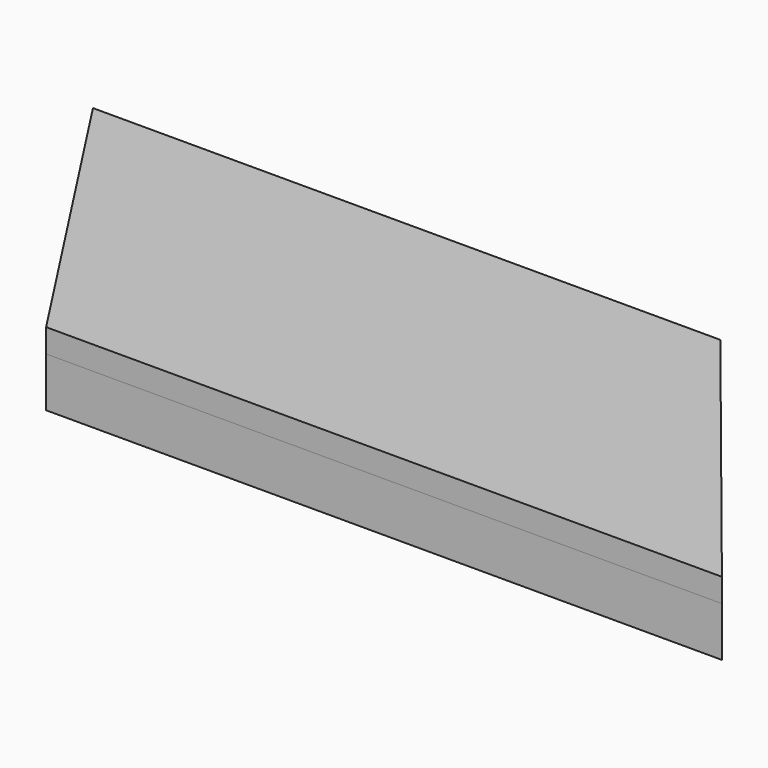
from build123d import *

# Parameters (mm, degrees)
F1_DEPTH = 2.54
F2_DEPTH = 2.794
F5_DEPTH = 2.54


# Not quite as in the source:
# - ends of sketch curves that miss each other by under 0.0002 mm in the source are joined


with BuildPart() as f1:
    # F0 (on Top) → F1 (new body)
    with BuildSketch(Plane.XY):
        Polygon((40.704589831, -14.0446320264), (45.6521262704, -14.1146421426), (31.6115576886, 3.3264026483), (26.7203815156, 3.3264026483), (24.2085343305, 6.4465921843), (-38.9784165732, 6.4465921843), (-22.1132018277, -19.5065848529), (45.1016274707, -19.5065848529), (43.1621550999, -17.0973931503), align=None)
        Polygon((26.7203815156, 3.3264026483), (31.6115576886, 3.3264026483), (26.0325449788, 10.2565921843), (-41.4542779326, 10.2565921843), (-38.9784165732, 6.4465921843), (24.2085343305, 6.4465921843), align=None)
        Polygon((53.0599689064, -23.3165845275), (49.0268522152, -18.3066903858), (45.6521262704, -14.1146421426), (40.704589831, -14.0446320264), (43.1621550999, -17.0973931503), (45.1016274707, -19.5065848529), (-22.1132018277, -19.5065848529), (-19.6373406798, -23.3165845275), align=None)
    extrude(amount=-F1_DEPTH)

    # F0 (on Top) → F2 (join)
    with BuildSketch(Plane.XY):
        Polygon((26.7203815156, 3.3264026483), (31.6115576886, 3.3264026483), (26.0325449788, 10.2565921843), (-41.4542779326, 10.2565921843), (-38.9784165732, 6.4465921843), (24.2085343305, 6.4465921843), align=None)
        Polygon((53.0599689064, -23.3165845275), (49.0268522152, -18.3066903858), (45.6521262704, -14.1146421426), (40.704589831, -14.0446320264), (43.1621550999, -17.0973931503), (45.1016274707, -19.5065848529), (-22.1132018277, -19.5065848529), (-19.6373406798, -23.3165845275), align=None)
    extrude(amount=F2_DEPTH)

    # F4 (on offset) → F5 (join)
    with BuildSketch(Plane.XY.offset(2.794)):
        Polygon((53.0598776368, -23.3175773174), (49.0267609456, -18.3076831757), (45.6520350008, -14.1156349324), (40.7044985614, -14.0456248163), (43.1620638303, -17.0983859402), (45.101536201, -19.5075776428), (-22.1132930973, -19.5075776428), (-19.6374319494, -23.3175773174), align=None)
        Polygon((40.7044985614, -14.0456248163), (45.6520350008, -14.1156349324), (31.611466419, 3.3254098585), (26.720290246, 3.3254098585), (24.2084430609, 6.4455993944), (-38.9785078428, 6.4455993944), (-22.1132930973, -19.5075776428), (45.101536201, -19.5075776428), (43.1620638303, -17.0983859402), align=None)
        Polygon((26.720290246, 3.3254098585), (31.611466419, 3.3254098585), (26.0324537092, 10.2555993944), (-41.4543692023, 10.2555993944), (-38.9785078428, 6.4455993944), (24.2084430609, 6.4455993944), align=None)
    extrude(amount=F5_DEPTH)


solid = f1.part
